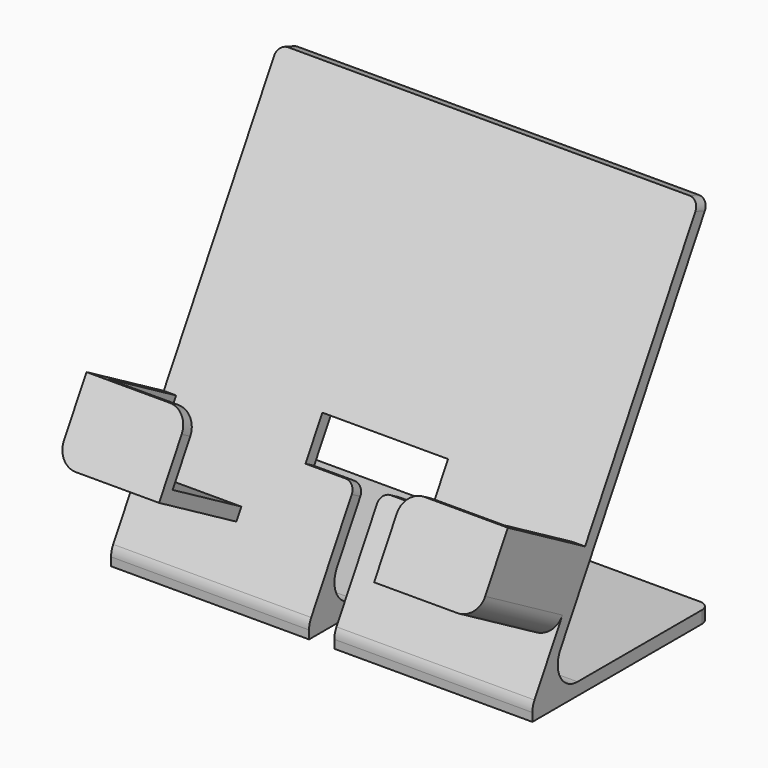
from build123d import *

# Parameters (mm, degrees)
F1_DEPTH = 53.975
F3_DEPTH = 25.4
F4_W     = 16.1045007408
F4_H     = 10.7811614871
F5_DEPTH = 3.175
F6_W     = 3.2399867196
F6_H     = 27.9691088945
F7_REACH = 124.3150351858
F8_W     = 26.4270068914
F8_H     = 19.5576284379
F9_DEPTH = 3.175
F10_R    = 5.08
F11_R    = 2.54


with BuildPart() as f1:
    # F0 (on Right) → F1 (new body)
    with BuildSketch(Plane.YZ):
        with BuildLine():
            Line((0, 0), (56.8904802203, 0))
            Line((56.8904802203, 0), (56.8904802203, 3.175))
            Line((56.8904802203, 3.175), (14.4803198381, 3.175))
            ThreePointArc((14.4803198381, 3.175), (8.981058524, 6.35), (8.981058524, 12.7))
            Line((8.981058524, 12.7), (56.5364878665, 95.0684197969))
            Line((56.5364878665, 95.0684197969), (53.4993190127, 96.1578890309))
            Line((53.4993190127, 96.1578890309), (0, 3.4943503306))
            Line((0, 3.4943503306), (0, 0))
        make_face()
    extrude(amount=F1_DEPTH)

    # F2 (on face) → F3 (join)
    with BuildSketch(Plane(origin=(0, -1.513098078, 0.8735875827), x_dir=(1, 0, 0), z_dir=(0, -0.8660254038, 0.5))):
        Polygon((27.5479931086, 17.2171894163), (53.975, 17.2171894163), (53.975, 36.7748178542), (50.8, 36.7748178542), (50.8, 20.3921894163), (27.5479931086, 20.3921894163), align=None)
    extrude(amount=F3_DEPTH)

    # F4 (on face) → F5 (cut, through all)
    with BuildSketch(Plane(origin=(0, -1.513098078, 0.8735875827), x_dir=(1, 0, 0), z_dir=(0, -0.8660254038, 0.5))):
        with Locations((8.0522503704, 38.3052378893)):
            Rectangle(F4_W, F4_H)
    extrude(amount=-F5_DEPTH, mode=Mode.SUBTRACT)

    f7_end = Plane(origin=(8.0522503704, 16.3190458234, 28.5847668277), x_dir=(0, 0.8660254038, -0.5), z_dir=(0, 0.5, 0.8660254038))
    # F6 (on Top) → F7 (cut, up to a plane its end follows)
    with BuildSketch(Plane.XY):
        with Locations((1.6199933598, 13.9845544472)):
            Rectangle(F6_W, F6_H)
    f7_long = extrude(amount=F7_REACH, mode=Mode.PRIVATE)
    add(split(f7_long, bisect_by=f7_end, keep=Keep.BOTTOM, mode=Mode.PRIVATE), mode=Mode.SUBTRACT)

    # F8 (on face) → F9 (join)
    with BuildSketch(Plane(origin=(0, -23.5101433341, 13.5735875827), x_dir=(1, 0, 0), z_dir=(0, -0.8660254038, 0.5))):
        with Locations((40.7614965543, 26.9960036352)):
            Rectangle(F8_W, F8_H)
    extrude(amount=F9_DEPTH)

    # F10
    f10_edges = [f1.edges().sort_by_distance(p)[0] for p in [
        (28.607493, 0, 3.49435),
        (53.975, -5.277841, 22.927861),
        (27.547993, -6.49755, 46.215264),
    ]]
    fillet(f10_edges, radius=F10_R)

    # F11
    f11_edges = [f1.edges().sort_by_distance(p)[0] for p in [
        (53.975, 55.017903, 95.613154),
        (53.975, 56.89048, 1.5875),
        (3.239987, 16.319046, 28.584767),
    ]]
    fillet(f11_edges, radius=F11_R)

    # F12: F1 across plane


with BuildPart() as f1_1:
    add(f1.part)
    add(f1.part.mirror(Plane.YZ))


solid = f1_1.part
